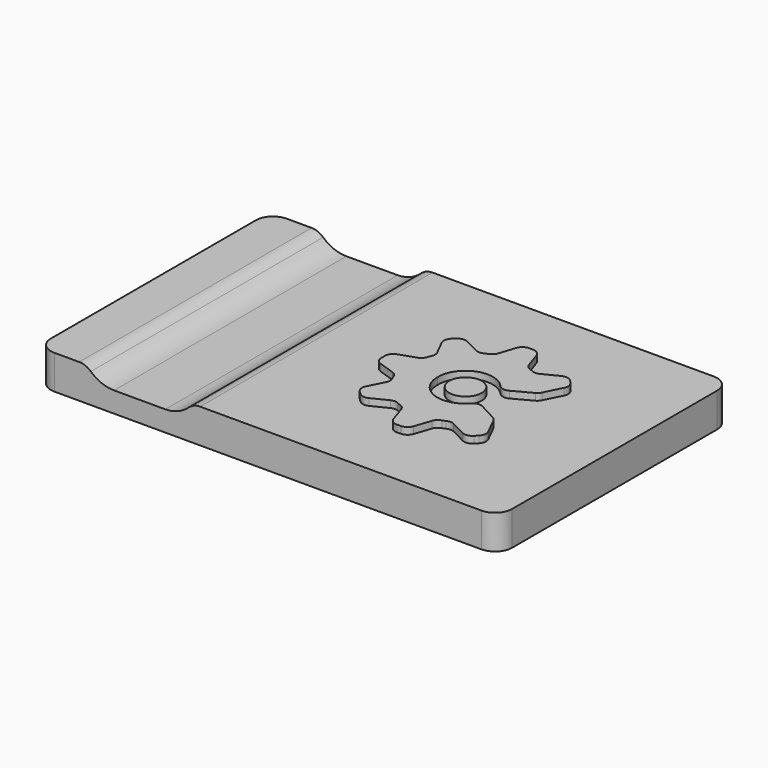
from build123d import *

# Parameters (mm, degrees)
F1_DEPTH = 6.35
F3_DEPTH = 76.2
F4_R     = 3.175
F6_DEPTH = 1.27
F5_R     = 3.022839237
F7_R     = 1.6002


with BuildPart() as f1:
    # F0 (on Top) → F1 (new body)
    with BuildSketch(Plane.XY):
        with BuildLine():
            Line((-39.6875, -26.9875), (39.6875, -26.9875))
            ThreePointArc((39.6875, -26.9875), (41.9325640303, -26.0575640303), (42.8625, -23.8125))
            Line((42.8625, -23.8125), (42.8625, 23.8125))
            ThreePointArc((42.8625, 23.8125), (41.9325640303, 26.0575640303), (39.6875, 26.9875))
            Line((39.6875, 26.9875), (-39.6875, 26.9875))
            ThreePointArc((-39.6875, 26.9875), (-41.9325640303, 26.0575640303), (-42.8625, 23.8125))
            Line((-42.8625, 23.8125), (-42.8625, -23.8125))
            ThreePointArc((-42.8625, -23.8125), (-41.9325640303, -26.0575640303), (-39.6875, -26.9875))
        make_face()
    extrude(amount=F1_DEPTH)

    # F2 (on face) → F3 (cut)
    with BuildSketch(Plane(origin=(0, 26.9875, 0), x_dir=(-1, 0, 0), z_dir=(0, 1, 0))):
        with BuildLine():
            ThreePointArc((19.05, 16.51), (12.7, 10.16), (19.05, 3.81))
            Line((19.05, 3.81), (28.575, 3.81))
            ThreePointArc((28.575, 3.81), (34.925, 10.16), (28.575, 16.51))
            Line((28.575, 16.51), (19.05, 16.51))
        make_face()
    extrude(amount=-F3_DEPTH, mode=Mode.SUBTRACT)

    # F4
    f4_edges = [f1.edges().sort_by_distance(p)[0] for p in [
        (-13.97, 0, 6.35),
        (-33.655, 0, 6.35),
    ]]
    fillet(f4_edges, radius=F4_R)

    # F5 (on face) → F6 (join)
    with BuildSketch(Plane.XY.offset(6.35)):
        with BuildLine():
            Line((26.9846954019, -9.8890943361), (24.6813038786, -5.2619308793))
            Line((24.6813038786, -5.2619308793), (19.6397530794, -2.5584178956))
            ThreePointArc((19.6397530794, -2.5584178956), (13.8718936075, -5.0986079783), (10.0536296353, -0.0844651021))
            ThreePointArc((10.0536296353, -0.0844651021), (13.8718936075, 4.929677774), (19.6397530794, 2.3894876914))
            Line((19.6397530794, 2.3894876914), (24.6813038786, 5.0930006751))
            Line((24.6813038786, 5.0930006751), (26.9846954019, 9.7201641319))
            Line((26.9846954019, 9.7201641319), (24.9206350104, 11.9179907053))
            Line((24.9206350104, 11.9179907053), (20.2478260164, 9.5458885687))
            ThreePointArc((20.2478260164, 9.5458885687), (19.3146437966, 10.0695514207), (18.2777250704, 10.3338455627))
            Line((18.2777250704, 10.3338455627), (16.6345701783, 15.2344879866))
            Line((16.6345701783, 15.2344879866), (13.6209610048, 15.3290749609))
            Line((13.6209610048, 15.3290749609), (11.9941155844, 10.3475705276))
            ThreePointArc((11.9941155844, 10.3475705276), (10.9639705549, 10.0579966056), (10.0438741121, 9.5116685229))
            Line((10.0438741121, 9.5116685229), (5.4167106552, 11.8150600462))
            Line((5.4167106552, 11.8150600462), (3.2188840818, 9.7509996548))
            Line((3.2188840818, 9.7509996548), (5.5909862184, 5.0781906607))
            ThreePointArc((5.5909862184, 5.0781906607), (5.0673233663, 4.1450084408), (4.8030292243, 3.1080897147))
            Line((4.8030292243, 3.1080897147), (-0.0976131995, 1.4649348226))
            Line((-0.0976131995, 1.4649348226), (-0.0976131995, -1.6338650268))
            Line((-0.0976131995, -1.6338650268), (4.8030292244, -3.2770199189))
            ThreePointArc((4.8030292244, -3.2770199189), (5.0673233664, -4.313938645), (5.5909862184, -5.2471208649))
            Line((5.5909862184, -5.2471208649), (3.2188840818, -9.919929859))
            Line((3.2188840818, -9.919929859), (5.4167106552, -11.9839902504))
            Line((5.4167106552, -11.9839902504), (10.0438741121, -9.6805987271))
            ThreePointArc((10.0438741121, -9.6805987271), (10.9639705549, -10.2269268099), (11.9941155844, -10.5165007319))
            Line((11.9941155844, -10.5165007319), (13.6209610048, -15.4980051652))
            Line((13.6209610048, -15.4980051652), (16.6345701783, -15.4034181908))
            Line((16.6345701783, -15.4034181908), (18.2777250704, -10.502775767))
            ThreePointArc((18.2777250704, -10.502775767), (19.3146437966, -10.238481625), (20.2478260164, -9.714818773))
            Line((20.2478260164, -9.714818773), (24.9206350104, -12.0869209095))
            Line((24.9206350104, -12.0869209095), (26.9846954019, -9.8890943361))
        make_face()
    extrude(amount=F6_DEPTH)

    # F7
    f7_edges = [f1.edges().sort_by_distance(p)[0] for p in [
        (3.218884, -9.91993, 6.985),
        (5.416711, -11.98399, 6.985),
        (10.043874, -9.680599, 6.985),
        (11.994116, -10.516501, 6.985),
        (13.620961, -15.498005, 6.985),
        (16.63457, -15.403418, 6.985),
        (24.920635, -12.086921, 6.985),
        (20.247826, -9.714819, 6.985),
        (18.277725, -10.502776, 6.985),
        (26.984695, -9.889094, 6.985),
        (24.681304, -5.261931, 6.985),
        (19.639753, -2.558418, 6.985),
        (19.639753, 2.389488, 6.985),
        (24.681304, 5.093001, 6.985),
        (26.984695, 9.720164, 6.985),
        (24.920635, 11.917991, 6.985),
        (20.247826, 9.545889, 6.985),
        (18.277725, 10.333846, 6.985),
        (16.63457, 15.234488, 6.985),
        (13.620961, 15.329075, 6.985),
        (11.994116, 10.347571, 6.985),
        (10.043874, 9.511669, 6.985),
        (5.416711, 11.81506, 6.985),
        (3.218884, 9.751, 6.985),
        (4.803029, 3.10809, 6.985),
        (5.590986, 5.078191, 6.985),
        (5.590986, -5.247121, 6.985),
        (4.803029, -3.27702, 6.985),
        (-0.097613, -1.633865, 6.985),
        (-0.097613, 1.464935, 6.985),
    ]]
    fillet(f7_edges, radius=F7_R)


with BuildPart() as f6:
    # F5 (on face) → F6, piece 2 (new body)
    with BuildSketch(Plane.XY.offset(6.35)):
        with Locations((15.1441273911, 0)):
            Circle(F5_R)
    extrude(amount=F6_DEPTH)


solid = Compound([f1.part, f6.part])
